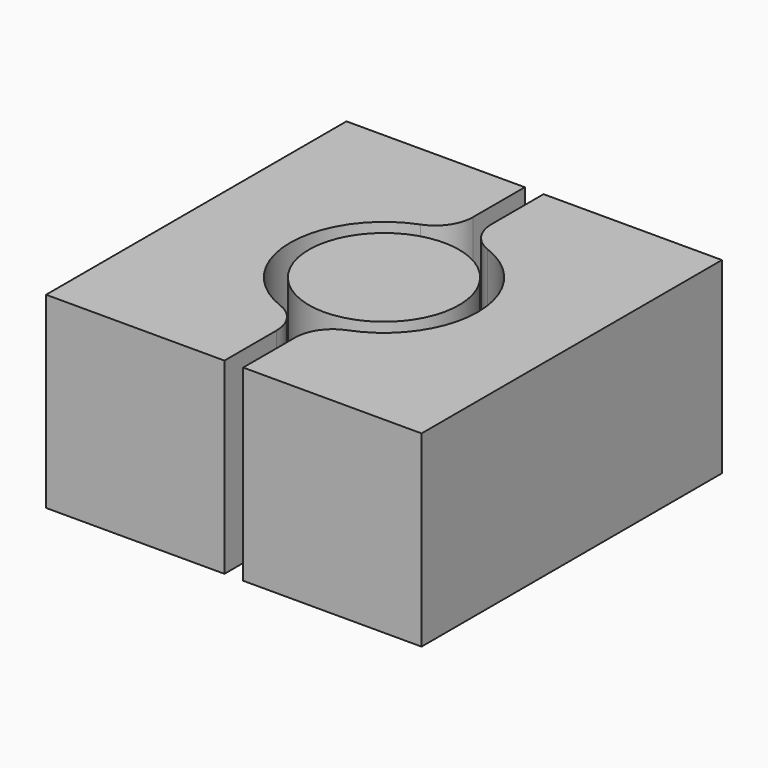
from build123d import *

# Parameters (mm, degrees)
F1_DEPTH = 5
F2_R     = 1
F2_2_R   = 1


# Not quite as in the source:
# - a feature names something its author has since deleted; it is built from what else it names


with BuildPart() as f1:
    # F0 (on Top) → F1 (new body)
    with BuildSketch(Plane.XY):
        with BuildLine():
            Line((5, -5), (5, 5))
            Line((5, 5), (0.25, 5))
            Line((0.25, 5), (0.25, 2.4874685928))
            ThreePointArc((0.25, 2.4874685928), (2.5, 0), (0.25, -2.4874685928))
            Line((0.25, -2.4874685928), (0.25, -5))
            Line((0.25, -5), (5, -5))
        make_face()
    extrude(amount=F1_DEPTH)

    # F2
    f2_edges = [f1.edges().sort_by_distance(p)[0] for p in [
        (0.25, -2.487469, 2.5),
        (0.25, 2.487469, 2.5),
    ]]
    fillet(f2_edges, radius=F2_R)


with BuildPart() as f1b:
    # F0 (on Top) → F1, piece 2 (new body)
    with BuildSketch(Plane.XY):
        with BuildLine():
            Line((-0.25, 5), (-5, 5))
            Line((-5, 5), (-5, -5))
            Line((-5, -5), (-0.25, -5))
            Line((-0.25, -5), (-0.25, -2.4874685928))
            ThreePointArc((-0.25, -2.4874685928), (-2.5, 0), (-0.25, 2.4874685928))
            Line((-0.25, 2.4874685928), (-0.25, 5))
        make_face()
    extrude(amount=F1_DEPTH)

    # F2#2
    f2_2_edges = [f1b.edges().sort_by_distance(p)[0] for p in [
        (-0.25, -2.487469, 2.5),
        (-0.25, 2.487469, 2.5),
    ]]
    fillet(f2_2_edges, radius=F2_2_R)


with BuildPart() as f1c:
    # F0 (on Top) → F1, piece 3 (new body)
    with BuildSketch(Plane.XY):
        with BuildLine():
            ThreePointArc((0, 2), (-2, 0), (0, -2))
            Line((0, -2), (0, 2))
        make_face()
        with BuildLine():
            Line((0, 2), (0, -2))
            ThreePointArc((0, -2), (2, 0), (0, 2))
        make_face()
    extrude(amount=F1_DEPTH)


solid = Compound([f1.part, f1b.part, f1c.part])
